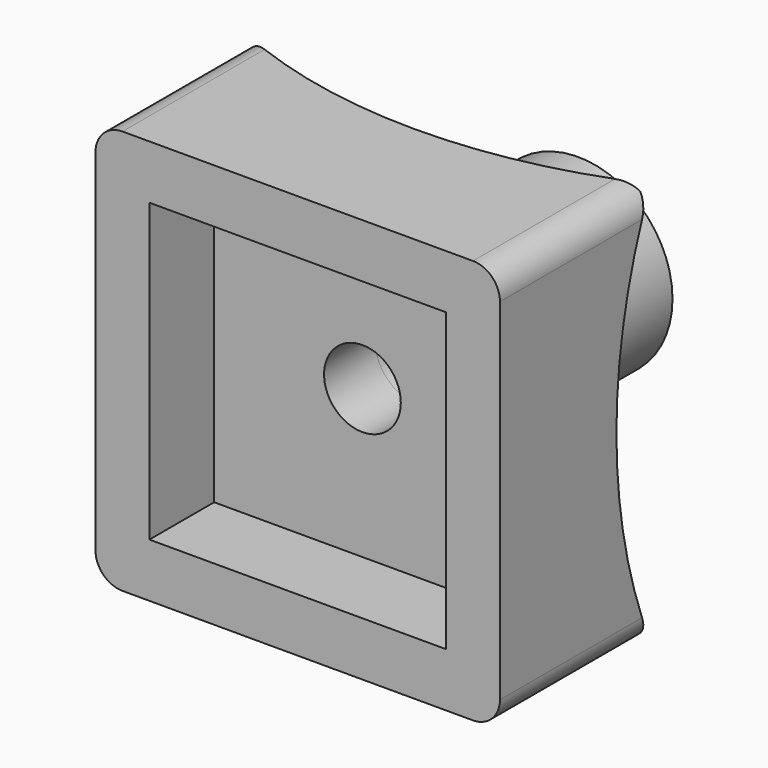
from build123d import *

# Parameters (mm, degrees)
F0_W      = 19.05
F0_H      = 19.05
F1_DEPTH  = 11.43
F3_DEPTH  = 19.051
F5_DEPTH  = 19.051
F6_R      = 4.445
F6_R_2    = 1.807104104
F7_DEPTH  = 19.05
F8_DEPTH  = 19.0510001
F9_W      = 2.54
F9_H      = 19.05
F10_DEPTH = 19.0510001
F11_W     = 13.97
F11_H     = 13.97
F11_R     = 4.445
F12_DEPTH = 6.35
F13_R     = 1.27


with BuildPart() as f1:
    # F0 (on Front) → F1 (new body)
    with BuildSketch(Plane.XZ):
        Rectangle(F0_W, F0_H)
    extrude(amount=F1_DEPTH)

    # F2 (on face) → F3 (cut, through all)
    with BuildSketch(Plane.YZ.offset(9.525)):
        with BuildLine():
            Line((0, -9.525), (0, 9.525))
            ThreePointArc((0, 9.525), (-2.032, 0), (0, -9.525))
        make_face()
    extrude(amount=-F3_DEPTH, mode=Mode.SUBTRACT)

    # F4 (on face) → F5 (cut, through all)
    with BuildSketch(Plane.XY.offset(9.525)):
        with BuildLine():
            ThreePointArc((9.525, 0), (19.5841950931, 8.6107735797), (23.34021875, 21.30821875))
            ThreePointArc((23.34021875, 21.30821875), (-12.6974451703, 40.8924138431), (-9.525, 0))
            Line((-9.525, 0), (9.525, 0))
        make_face()
        with BuildLine():
            Line((9.525, 0), (-9.525, 0))
            ThreePointArc((-9.525, 0), (0, -2.032), (9.525, 0))
        make_face()
    extrude(amount=-F5_DEPTH, mode=Mode.SUBTRACT)

    # F6 (on face) → F7 (join)
    with BuildSketch(Plane.XZ.offset(11.43)):
        Circle(F6_R)
        Circle(F6_R_2, mode=Mode.SUBTRACT)
    extrude(amount=-F7_DEPTH)

    # F6 (on face) → F8 (cut, through all)
    with BuildSketch(Plane.XZ.offset(11.43)):
        Circle(F6_R_2)
    extrude(amount=-F8_DEPTH, mode=Mode.SUBTRACT)

    # F9 (on face) → F10 (cut, through all)
    with BuildSketch(Plane.YZ.offset(9.525)):
        with Locations((-10.16, 0)):
            Rectangle(F9_W, F9_H)
    extrude(amount=-F10_DEPTH, mode=Mode.SUBTRACT)

    # F11 (on face) + F6 (on face) → F12 (cut)
    with BuildSketch(Plane.XZ.offset(11.43)):
        Rectangle(F11_W, F11_H)
        Circle(F11_R, mode=Mode.SUBTRACT)
    with BuildSketch(Plane.XZ.offset(11.43)):
        Circle(F6_R)
        Circle(F6_R_2, mode=Mode.SUBTRACT)
    extrude(amount=-F12_DEPTH, mode=Mode.SUBTRACT)

    # F13
    f13_edges = [f1.edges().sort_by_distance(p)[0] for p in [
        (-9.525, -4.445, -9.525),
        (-9.525, -4.445, 9.525),
        (9.525, -4.445, 9.525),
        (9.525, -4.445, -9.525),
    ]]
    fillet(f13_edges, radius=F13_R)


solid = f1.part
